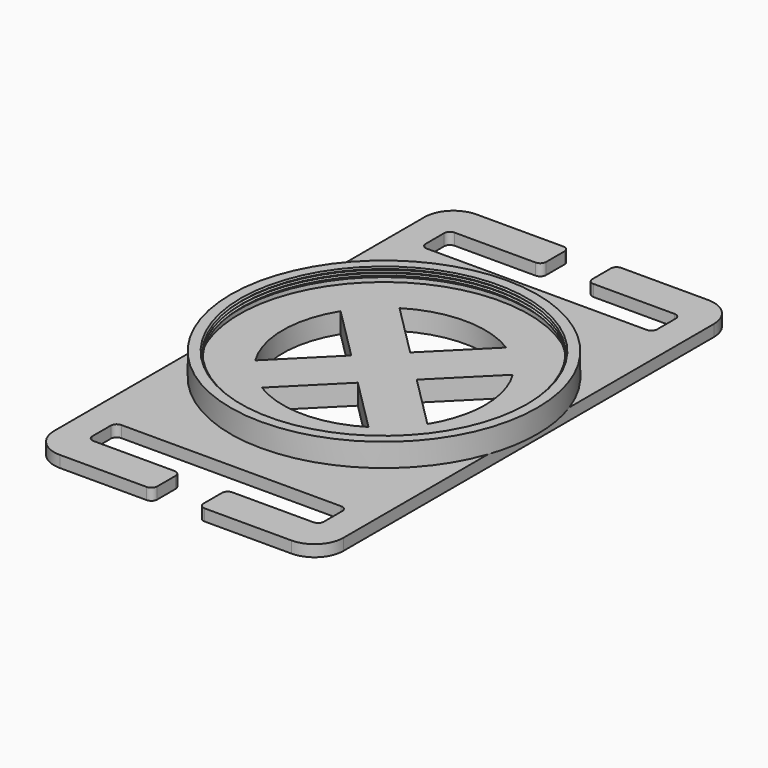
from build123d import *

# Parameters (mm, degrees)
F0_W      = 50
F0_H      = 90
F1_DEPTH  = 2
F2_R      = 26.5
F3_DEPTH  = 1.5
F4_R      = 26.5
F4_R_2    = 25
F5_DEPTH  = 1
F6_W      = 3
F6_H      = 70
F7_DEPTH  = 3
F8_DEPTH  = 3
F10_DEPTH = 25
F11_W     = 8
F11_H     = 6
F12_DEPTH = 25
F13_R     = 1
F14_R     = 1
F15_R     = 5
F18_SIZE  = 0.25
F19_R     = 26.5
F19_R_2   = 25.25
F19_R_3   = 24.5
F20_DEPTH = 0.5
F21_SIZE  = 0.24999
F22_R     = 26.5
F22_R_2   = 24.74999
F22_R_3   = 24.5
F23_DEPTH = 0.5
F24_SIZE  = 0.2499
F25_R     = 26.5
F25_R_2   = 24.7499
F25_R_3   = 24.5
F26_DEPTH = 0.5
F27_SIZE  = 0.249


# Not quite as in the source:
# - a fillet or chamfer is up to 0.001 mm smaller than in the source, because OpenCascade refuses the exact size


with BuildPart() as f1:
    # F0 (on Top) → F1 (new body)
    with BuildSketch(Plane.XY):
        Rectangle(F0_W, F0_H)
    extrude(amount=F1_DEPTH)

    # F2 (on face) → F3 (join)
    with BuildSketch(Plane.XY.offset(2)):
        Circle(F2_R)
    extrude(amount=F3_DEPTH)

    # F4 (on face) → F5 (join)
    with BuildSketch(Plane.XY.offset(3.5)):
        Circle(F4_R)
        Circle(F4_R_2, mode=Mode.SUBTRACT)
    extrude(amount=F5_DEPTH)

    # F6 (on face) → F7 (join)
    with BuildSketch(Plane(origin=(0, 0, 0), x_dir=(1, 0, 0), z_dir=(0, 0, -1))):
        with Locations((-23.5, 0)):
            Rectangle(F6_W, F6_H)
        with Locations((23.5, 0)):
            Rectangle(F6_W, F6_H)
    extrude(amount=F7_DEPTH)

    # F8 (cut, through all): faces of the model
    f8_faces = [f1.faces().sort_by_distance(p)[0] for p in [
        (-23.5, 0, -3),
        (23.5, 0, -3),
        (-23.5, 0, -3),
        (23.5, 0, -3),
    ]]
    extrude(f8_faces, amount=-F8_DEPTH, mode=Mode.SUBTRACT)

    # F9 (on face) → F10 (cut)
    with BuildSketch(Plane.XY.offset(3.5)):
        with BuildLine():
            Line((-5.6568542495, 0), (-14.8752109279, 9.2183566784))
            ThreePointArc((-14.8752109279, 9.2183566784), (-17.5, 0), (-14.8752109279, -9.2183566784))
            Line((-14.8752109279, -9.2183566784), (-5.6568542495, 0))
        make_face()
        with BuildLine():
            ThreePointArc((-9.2183566784, -14.8752109279), (0, -17.5), (9.2183566784, -14.8752109279))
            Line((9.2183566784, -14.8752109279), (0, -5.6568542495))
            Line((0, -5.6568542495), (-9.2183566784, -14.8752109279))
        make_face()
        with BuildLine():
            ThreePointArc((14.8752109279, -9.2183566784), (16.831015882, -4.7923798244), (17.5, 0))
            ThreePointArc((17.5, 0), (16.831015882, 4.7923798244), (14.8752109279, 9.2183566784))
            Line((14.8752109279, 9.2183566784), (5.6568542495, 0))
            Line((5.6568542495, 0), (14.8752109279, -9.2183566784))
        make_face()
        with BuildLine():
            Line((0, 5.6568542495), (9.2183566784, 14.8752109279))
            ThreePointArc((9.2183566784, 14.8752109279), (0, 17.5), (-9.2183566784, 14.8752109279))
            Line((-9.2183566784, 14.8752109279), (0, 5.6568542495))
        make_face()
    extrude(amount=-F10_DEPTH, mode=Mode.SUBTRACT)

    # F11 (on face) → F12 (cut)
    with BuildSketch(Plane(origin=(0, 0, 0), x_dir=(1, 0, 0), z_dir=(0, 0, -1))):
        with Locations((0, -42)):
            Rectangle(F11_W, F11_H)
        with BuildLine():
            Line((-4, -39), (4, -39))
            Line((4, -39), (19, -39))
            ThreePointArc((19, -39), (19.7071067812, -38.7071067812), (20, -38))
            Line((20, -38), (20, -34))
            ThreePointArc((20, -34), (19.7071067812, -33.2928932188), (19, -33))
            Line((19, -33), (-19, -33))
            ThreePointArc((-19, -33), (-19.7071067812, -33.2928932188), (-20, -34))
            Line((-20, -34), (-20, -38))
            ThreePointArc((-20, -38), (-19.7071067812, -38.7071067812), (-19, -39))
            Line((-19, -39), (-4, -39))
        make_face()
        with Locations((0, 42)):
            Rectangle(F11_W, F11_H)
        with BuildLine():
            ThreePointArc((20, 38), (19.7071067812, 38.7071067812), (19, 39))
            Line((19, 39), (4, 39))
            Line((4, 39), (-4, 39))
            Line((-4, 39), (-19, 39))
            ThreePointArc((-19, 39), (-19.7071067812, 38.7071067812), (-20, 38))
            Line((-20, 38), (-20, 34))
            ThreePointArc((-20, 34), (-19.7071067812, 33.2928932188), (-19, 33))
            Line((-19, 33), (19, 33))
            ThreePointArc((19, 33), (19.7071067812, 33.2928932188), (20, 34))
            Line((20, 34), (20, 38))
        make_face()
    extrude(amount=-F12_DEPTH, mode=Mode.SUBTRACT)

    # F13
    f13_edges = [f1.edges().sort_by_distance(p)[0] for p in [
        (-4, -45, 1),
        (-4, -39, 1),
        (4, -45, 1),
        (4, -39, 1),
    ]]
    fillet(f13_edges, radius=F13_R)

    # F14
    f14_edges = [f1.edges().sort_by_distance(p)[0] for p in [
        (4, 45, 1),
        (4, 39, 1),
        (-4, 45, 1),
        (-4, 39, 1),
    ]]
    fillet(f14_edges, radius=F14_R)

    # F15
    f15_edges = [f1.edges().sort_by_distance(p)[0] for p in [
        (25, -45, 1),
        (25, 45, 1),
        (-25, 45, 1),
        (-25, -45, 1),
    ]]
    fillet(f15_edges, radius=F15_R)


with BuildPart() as f16_1:
    # F16: copy of F1
    add(f1.part.moved(Location((72.1, 0, 0))))


with BuildPart() as f1_1:
    add(f1.part)

    # F18
    f18_edges = [f1_1.edges().sort_by_distance(p)[0] for p in [
        (-25, 0, 4.5),
    ]]
    chamfer(f18_edges, length=F18_SIZE)

    # F19 (on face) → F20 (join)
    with BuildSketch(Plane.XY.offset(4.5)):
        Circle(F19_R)
        Circle(F19_R_2, mode=Mode.SUBTRACT)
        Circle(F19_R_2)
        Circle(F19_R_3, mode=Mode.SUBTRACT)
    extrude(amount=F20_DEPTH)

    # F21 (size 0.25 in the source; OpenCascade refuses exactly that, so slightly less here)
    f21_edges = [f1_1.edges().sort_by_distance(p)[0] for p in [
        (-24.5, 0, 4.5),
        (-24.5, 0, 5),
    ]]
    chamfer(f21_edges, length=F21_SIZE)

    # F22 (on face) → F23 (join)
    with BuildSketch(Plane.XY.offset(5)):
        Circle(F22_R)
        Circle(F22_R_2, mode=Mode.SUBTRACT)
        Circle(F22_R_2)
        Circle(F22_R_3, mode=Mode.SUBTRACT)
    extrude(amount=F23_DEPTH)

    # F24 (size 0.25 in the source; OpenCascade refuses exactly that, so slightly less here)
    f24_edges = [f1_1.edges().sort_by_distance(p)[0] for p in [
        (-24.5, 0, 5),
        (-24.5, 0, 5.5),
    ]]
    chamfer(f24_edges, length=F24_SIZE)

    # F25 (on face) → F26 (join)
    with BuildSketch(Plane.XY.offset(5.5)):
        Circle(F25_R)
        Circle(F25_R_2, mode=Mode.SUBTRACT)
        Circle(F25_R_2)
        Circle(F25_R_3, mode=Mode.SUBTRACT)
    extrude(amount=F26_DEPTH)

    # F27 (size 0.25 in the source; OpenCascade refuses exactly that, so slightly less here)
    f27_edges = [f1_1.edges().sort_by_distance(p)[0] for p in [
        (-24.5, 0, 6),
        (-24.5, 0, 5.5),
    ]]
    chamfer(f27_edges, length=F27_SIZE)


solid = f1_1.part
